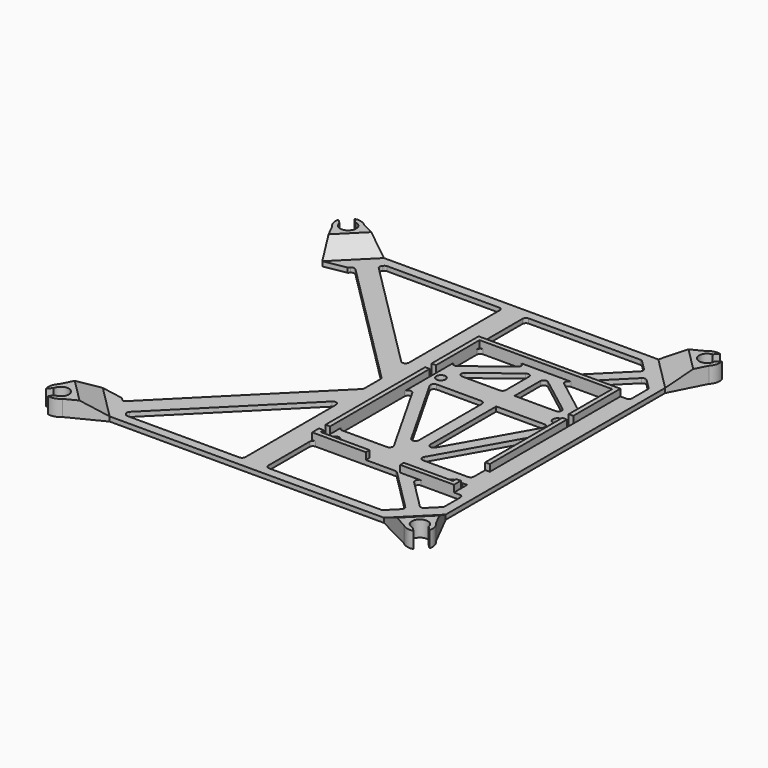
from build123d import *

# Parameters (mm, degrees)
F0_W          = 150
F0_H          = 150
F1_DEPTH      = 2
F2_W          = 62
F2_H          = 91
F2_W_2        = 58
F2_H_2        = 87
F3_DEPTH      = 3
F4_W          = 15
F4_H          = 2
F4_W_2        = 2
F4_H_2        = 14
F5_DEPTH      = 3
F6_R          = 2
F6_W          = 2
F6_H          = 3.5
F7_DEPTH      = 25
F9_DEPTH      = 5
F9_DEPTH_BACK = 2
F10_DEPTH     = 5
F11_DEPTH     = 5
F12_SIZE2     = 4.99999
F12_SIZE      = 9.99999
F12_2_SIZE2   = 4.99999
F12_2_SIZE    = 9.99999
F12_3_SIZE2   = 4.99999
F12_3_SIZE    = 9.99999
F12_4_SIZE2   = 4.99999
F12_4_SIZE    = 9.99999
F14_DEPTH     = 25
F16_DEPTH     = 25
F17_R         = 1.5
F18_R         = 1.5
F19_R         = 1.5
F21_R         = 1
F23_DEPTH     = 25
F25_DEPTH     = 25


# Not quite as in the source:
# - two fillets or chamfers of one size are made in one step
# - a fillet or chamfer is up to 0.001 mm smaller than in the source, because OpenCascade refuses the exact size


with BuildPart() as f1:
    # F0 (on Top) → F1 (new body)
    with BuildSketch(Plane.XY):
        Rectangle(F0_W, F0_H)
    extrude(amount=F1_DEPTH)

    # F2 (on face) → F3 (join)
    with BuildSketch(Plane.XY.offset(2)):
        with Locations((36, 0)):
            Rectangle(F2_W, F2_H)
        with Locations((36, 0)):
            Rectangle(F2_W_2, F2_H_2, mode=Mode.SUBTRACT)
    extrude(amount=F3_DEPTH)

    # F4 (on face) → F5 (cut)
    with BuildSketch(Plane.XY.offset(5)):
        with Locations((36, -44.5)):
            Rectangle(F4_W, F4_H)
        with Locations((66, -32.9)):
            Rectangle(F4_W_2, F4_H_2)
    extrude(amount=-F5_DEPTH, mode=Mode.SUBTRACT)

    # F6 (on face) → F7 (cut)
    with BuildSketch(Plane.XY.offset(5)):
        with Locations((61.5, -40)):
            Circle(F6_R)
        with Locations((61.5, 18)):
            Circle(F6_R)
        with Locations((66, -40)):
            Rectangle(F6_W, F6_H)
        with Locations((66, 18)):
            Rectangle(F6_W, F6_H)
        with Locations((6, -40)):
            Rectangle(F6_W, F6_H)
        with Locations((6, 18)):
            Rectangle(F6_W, F6_H)
        with Locations((10.5, 18)):
            Circle(F6_R)
        with Locations((10.5, -40)):
            Circle(F6_R)
    extrude(amount=-F7_DEPTH, mode=Mode.SUBTRACT)

    # F8 (on face) → F9 (join, two sides)
    with BuildSketch(Plane.XY.offset(2)) as f9_sk:
        with BuildLine():
            ThreePointArc((82.0110086434, 78.1219213469), (76.0606601718, 76.0606601718), (78.1219213469, 82.0110086434))
            Line((78.1219213469, 82.0110086434), (79.959038654, 83.8481259505))
            ThreePointArc((79.959038654, 83.8481259505), (77.1120291579, 83.8481259505), (74.6464466094, 82.4246212025))
            Line((74.6464466094, 82.4246212025), (60, 75))
            Line((60, 75), (75, 60))
            Line((75, 60), (82.4246212025, 74.6464466094))
            ThreePointArc((82.4246212025, 74.6464466094), (83.8481259505, 77.1120291579), (83.8481259505, 79.959038654))
            Line((83.8481259505, 79.959038654), (82.0110086434, 78.1219213469))
        make_face()
        with BuildLine():
            Line((-60, 75), (-74.6464466094, 82.4246212025))
            ThreePointArc((-74.6464466094, 82.4246212025), (-77.1120291579, 83.8481259505), (-79.959038654, 83.8481259505))
            Line((-79.959038654, 83.8481259505), (-78.1219213469, 82.0110086434))
            ThreePointArc((-78.1219213469, 82.0110086434), (-76.0606601718, 76.0606601718), (-82.0110086434, 78.1219213469))
            Line((-82.0110086434, 78.1219213469), (-83.8481259505, 79.959038654))
            ThreePointArc((-83.8481259505, 79.959038654), (-83.8481259505, 77.1120291579), (-82.4246212025, 74.6464466094))
            Line((-82.4246212025, 74.6464466094), (-75, 60))
            Line((-75, 60), (-60, 75))
        make_face()
        with BuildLine():
            Line((-75, -60), (-82.4246212025, -74.6464466094))
            ThreePointArc((-82.4246212025, -74.6464466094), (-83.8481259505, -77.1120291579), (-83.8481259505, -79.959038654))
            Line((-83.8481259505, -79.959038654), (-82.0110086434, -78.1219213469))
            ThreePointArc((-82.0110086434, -78.1219213469), (-76.0606601718, -76.0606601718), (-78.1219213469, -82.0110086434))
            Line((-78.1219213469, -82.0110086434), (-79.959038654, -83.8481259505))
            ThreePointArc((-79.959038654, -83.8481259505), (-77.1120291579, -83.8481259505), (-74.6464466094, -82.4246212025))
            Line((-74.6464466094, -82.4246212025), (-60, -75))
            Line((-60, -75), (-75, -60))
        make_face()
        with BuildLine():
            Line((60, -75), (74.6464466094, -82.4246212025))
            ThreePointArc((74.6464466094, -82.4246212025), (77.1120291579, -83.8481259505), (79.959038654, -83.8481259505))
            Line((79.959038654, -83.8481259505), (78.1219213469, -82.0110086434))
            ThreePointArc((78.1219213469, -82.0110086434), (76.0606601718, -76.0606601718), (82.0110086434, -78.1219213469))
            Line((82.0110086434, -78.1219213469), (83.8481259505, -79.959038654))
            ThreePointArc((83.8481259505, -79.959038654), (83.8481259505, -77.1120291579), (82.4246212025, -74.6464466094))
            Line((82.4246212025, -74.6464466094), (75, -60))
            Line((75, -60), (60, -75))
        make_face()
    extrude(amount=F9_DEPTH)
    extrude(f9_sk.sketch, amount=-F9_DEPTH_BACK)

    # F8 (on face) → F10 (join)
    with BuildSketch(Plane.XY.offset(2)):
        with BuildLine():
            ThreePointArc((82.0110086434, 78.1219213469), (76.0606601718, 76.0606601718), (78.1219213469, 82.0110086434))
            Line((78.1219213469, 82.0110086434), (79.959038654, 83.8481259505))
            ThreePointArc((79.959038654, 83.8481259505), (77.1120291579, 83.8481259505), (74.6464466094, 82.4246212025))
            Line((74.6464466094, 82.4246212025), (60, 75))
            Line((60, 75), (75, 60))
            Line((75, 60), (82.4246212025, 74.6464466094))
            ThreePointArc((82.4246212025, 74.6464466094), (83.8481259505, 77.1120291579), (83.8481259505, 79.959038654))
            Line((83.8481259505, 79.959038654), (82.0110086434, 78.1219213469))
        make_face()
        with BuildLine():
            Line((-60, 75), (-74.6464466094, 82.4246212025))
            ThreePointArc((-74.6464466094, 82.4246212025), (-77.1120291579, 83.8481259505), (-79.959038654, 83.8481259505))
            Line((-79.959038654, 83.8481259505), (-78.1219213469, 82.0110086434))
            ThreePointArc((-78.1219213469, 82.0110086434), (-76.0606601718, 76.0606601718), (-82.0110086434, 78.1219213469))
            Line((-82.0110086434, 78.1219213469), (-83.8481259505, 79.959038654))
            ThreePointArc((-83.8481259505, 79.959038654), (-83.8481259505, 77.1120291579), (-82.4246212025, 74.6464466094))
            Line((-82.4246212025, 74.6464466094), (-75, 60))
            Line((-75, 60), (-60, 75))
        make_face()
        with BuildLine():
            Line((-75, -60), (-82.4246212025, -74.6464466094))
            ThreePointArc((-82.4246212025, -74.6464466094), (-83.8481259505, -77.1120291579), (-83.8481259505, -79.959038654))
            Line((-83.8481259505, -79.959038654), (-82.0110086434, -78.1219213469))
            ThreePointArc((-82.0110086434, -78.1219213469), (-76.0606601718, -76.0606601718), (-78.1219213469, -82.0110086434))
            Line((-78.1219213469, -82.0110086434), (-79.959038654, -83.8481259505))
            ThreePointArc((-79.959038654, -83.8481259505), (-77.1120291579, -83.8481259505), (-74.6464466094, -82.4246212025))
            Line((-74.6464466094, -82.4246212025), (-60, -75))
            Line((-60, -75), (-75, -60))
        make_face()
        with BuildLine():
            Line((60, -75), (74.6464466094, -82.4246212025))
            ThreePointArc((74.6464466094, -82.4246212025), (77.1120291579, -83.8481259505), (79.959038654, -83.8481259505))
            Line((79.959038654, -83.8481259505), (78.1219213469, -82.0110086434))
            ThreePointArc((78.1219213469, -82.0110086434), (76.0606601718, -76.0606601718), (82.0110086434, -78.1219213469))
            Line((82.0110086434, -78.1219213469), (83.8481259505, -79.959038654))
            ThreePointArc((83.8481259505, -79.959038654), (83.8481259505, -77.1120291579), (82.4246212025, -74.6464466094))
            Line((82.4246212025, -74.6464466094), (75, -60))
            Line((75, -60), (60, -75))
        make_face()
    extrude(amount=F10_DEPTH)

    # F8 (on face) → F11 (join)
    with BuildSketch(Plane.XY.offset(2)):
        with BuildLine():
            ThreePointArc((82.0110086434, 78.1219213469), (76.0606601718, 76.0606601718), (78.1219213469, 82.0110086434))
            Line((78.1219213469, 82.0110086434), (79.959038654, 83.8481259505))
            ThreePointArc((79.959038654, 83.8481259505), (77.1120291579, 83.8481259505), (74.6464466094, 82.4246212025))
            Line((74.6464466094, 82.4246212025), (60, 75))
            Line((60, 75), (75, 60))
            Line((75, 60), (82.4246212025, 74.6464466094))
            ThreePointArc((82.4246212025, 74.6464466094), (83.8481259505, 77.1120291579), (83.8481259505, 79.959038654))
            Line((83.8481259505, 79.959038654), (82.0110086434, 78.1219213469))
        make_face()
        with BuildLine():
            Line((-60, 75), (-74.6464466094, 82.4246212025))
            ThreePointArc((-74.6464466094, 82.4246212025), (-77.1120291579, 83.8481259505), (-79.959038654, 83.8481259505))
            Line((-79.959038654, 83.8481259505), (-78.1219213469, 82.0110086434))
            ThreePointArc((-78.1219213469, 82.0110086434), (-76.0606601718, 76.0606601718), (-82.0110086434, 78.1219213469))
            Line((-82.0110086434, 78.1219213469), (-83.8481259505, 79.959038654))
            ThreePointArc((-83.8481259505, 79.959038654), (-83.8481259505, 77.1120291579), (-82.4246212025, 74.6464466094))
            Line((-82.4246212025, 74.6464466094), (-75, 60))
            Line((-75, 60), (-60, 75))
        make_face()
        with BuildLine():
            Line((-75, -60), (-82.4246212025, -74.6464466094))
            ThreePointArc((-82.4246212025, -74.6464466094), (-83.8481259505, -77.1120291579), (-83.8481259505, -79.959038654))
            Line((-83.8481259505, -79.959038654), (-82.0110086434, -78.1219213469))
            ThreePointArc((-82.0110086434, -78.1219213469), (-76.0606601718, -76.0606601718), (-78.1219213469, -82.0110086434))
            Line((-78.1219213469, -82.0110086434), (-79.959038654, -83.8481259505))
            ThreePointArc((-79.959038654, -83.8481259505), (-77.1120291579, -83.8481259505), (-74.6464466094, -82.4246212025))
            Line((-74.6464466094, -82.4246212025), (-60, -75))
            Line((-60, -75), (-75, -60))
        make_face()
        with BuildLine():
            Line((60, -75), (74.6464466094, -82.4246212025))
            ThreePointArc((74.6464466094, -82.4246212025), (77.1120291579, -83.8481259505), (79.959038654, -83.8481259505))
            Line((79.959038654, -83.8481259505), (78.1219213469, -82.0110086434))
            ThreePointArc((78.1219213469, -82.0110086434), (76.0606601718, -76.0606601718), (82.0110086434, -78.1219213469))
            Line((82.0110086434, -78.1219213469), (83.8481259505, -79.959038654))
            ThreePointArc((83.8481259505, -79.959038654), (83.8481259505, -77.1120291579), (82.4246212025, -74.6464466094))
            Line((82.4246212025, -74.6464466094), (75, -60))
            Line((75, -60), (60, -75))
        make_face()
    extrude(amount=F11_DEPTH)

    # F12 (size 10 and 5 in the source; OpenCascade refuses exactly that, so slightly less here)
    f12_edges = [f1.edges().sort_by_distance(p)[0] for p in [
        (-67.5, 67.5, 7),
    ]]
    f12_side = f1.faces().sort_by_distance((-72.538706, 72.538706, 7))[0]
    chamfer(f12_edges, length=F12_SIZE, length2=F12_SIZE2, reference=f12_side)

    # F12#2 (size 10 and 5 in the source; OpenCascade refuses exactly that, so slightly less here)
    f12_2_edges = [f1.edges().sort_by_distance(p)[0] for p in [
        (67.5, 67.5, 7),
    ]]
    f12_2_side = f1.faces().sort_by_distance((72.538706, 72.538706, 7))[0]
    chamfer(f12_2_edges, length=F12_2_SIZE, length2=F12_2_SIZE2, reference=f12_2_side)

    # F12#3 (size 10 and 5 in the source; OpenCascade refuses exactly that, so slightly less here)
    f12_3_edges = [f1.edges().sort_by_distance(p)[0] for p in [
        (67.5, -67.5, 7),
    ]]
    f12_3_side = f1.faces().sort_by_distance((72.538706, -72.538706, 7))[0]
    chamfer(f12_3_edges, length=F12_3_SIZE, length2=F12_3_SIZE2, reference=f12_3_side)

    # F12#4 (size 10 and 5 in the source; OpenCascade refuses exactly that, so slightly less here)
    f12_4_edges = [f1.edges().sort_by_distance(p)[0] for p in [
        (-67.5, -67.5, 7),
    ]]
    f12_4_side = f1.faces().sort_by_distance((-72.538706, -72.538706, 7))[0]
    chamfer(f12_4_edges, length=F12_4_SIZE, length2=F12_4_SIZE2, reference=f12_4_side)

    # F13 (on face) → F14 (cut)
    with BuildSketch(Plane.XY.offset(2)):
        with BuildLine():
            ThreePointArc((-7.5606601718, 18.8743686708), (-5.9259748515, 18.5492095438), (-5, 19.9350288425))
            Line((-5, 19.9350288425), (-5, 71))
            Line((-5, 71), (-56, 71))
            Line((-56, 71), (-56.7824855787, 70.2175144213))
            ThreePointArc((-56.7824855787, 70.2175144213), (-57.2218254069, 69.1568542495), (-56.7824855787, 68.0961940777))
            Line((-56.7824855787, 68.0961940777), (-7.5606601718, 18.8743686708))
        make_face()
        Polygon((56, 71), (5, 71), (5, 45.5), (41.9644660941, 45.5), (61.732233047, 65.267766953), align=None)
        Polygon((67, -45.5), (49.0355339059, -45.5), (65.267766953, -61.732233047), (71, -56), (71, -45.5), align=None)
        Polygon((-5, -71), (-5, -16.313708499), (-57.8431457505, -69.1568542495), (-56, -71), align=None)
        Polygon((41.9644660941, -45.5), (5, -45.5), (5, -71), (56, -71), (61.732233047, -65.267766953), align=None)
        Polygon((-65.267766953, 61.732233047), (-71, 56), (-71, 5), (-71, -5), (-5, -5), (-5, 5), (-63.5, 63.5), align=None)
        Polygon((-5, -5), (-71, -5), (-71, -56), (-65.267766953, -61.732233047), (-63.5, -63.5), align=None)
        Polygon((65.267766953, 61.732233047), (49.0355339059, 45.5), (67, 45.5), (71, 45.5), (71, 56), align=None)
    extrude(amount=-F14_DEPTH, mode=Mode.SUBTRACT)

    # F15 (on face) → F16 (cut)
    with BuildSketch(Plane.XY.offset(5)):
        with BuildLine():
            Line((33.5, -22.7423213834), (33.5, 11.75))
            ThreePointArc((33.5, 11.75), (33.0606601718, 12.8106601718), (32, 13.25))
            Line((32, 13.25), (12.4482028522, 13.25))
            ThreePointArc((12.4482028522, 13.25), (11.1521429804, 12.5051349607), (11.1432693585, 11.0103050784))
            Line((11.1432693585, 11.0103050784), (30.6950665063, -23.482016305))
            ThreePointArc((30.6950665063, -23.482016305), (32.3824916727, -24.1927351589), (33.5, -22.7423213834))
        make_face()
        with BuildLine():
            ThreePointArc((25.8598739427, 40.808144173), (26.3699933362, 42.4807370692), (24.949116188, 43.5))
            Line((24.949116188, 43.5), (8.5, 43.5))
            ThreePointArc((8.5, 43.5), (7.4393398282, 43.0606601718), (7, 42))
            Line((7, 42), (7, 29.4303923469))
            ThreePointArc((7, 29.4303923469), (7.8352205749, 28.0857480385), (9.4107577546, 28.2385365198))
            Line((9.4107577546, 28.2385365198), (25.8598739427, 40.808144173))
        make_face()
        with BuildLine():
            ThreePointArc((60.8567306415, 11.0103050784), (60.8478570196, 12.5051349607), (59.5517971478, 13.25))
            Line((59.5517971478, 13.25), (40, 13.25))
            ThreePointArc((40, 13.25), (38.9393398282, 12.8106601718), (38.5, 11.75))
            Line((38.5, 11.75), (38.5, -22.7423213834))
            ThreePointArc((38.5, -22.7423213834), (39.6175083273, -24.1927351589), (41.3049334937, -23.482016305))
            Line((41.3049334937, -23.482016305), (60.8567306415, 11.0103050784))
        make_face()
        with BuildLine():
            ThreePointArc((33.5, 37.3196076531), (32.6647794251, 38.6642519615), (31.0892422454, 38.5114634802))
            Line((31.0892422454, 38.5114634802), (14.6401260573, 25.941855827))
            ThreePointArc((14.6401260573, 25.941855827), (14.1300066638, 24.2692629308), (15.550883812, 23.25))
            Line((15.550883812, 23.25), (32, 23.25))
            ThreePointArc((32, 23.25), (33.0606601718, 23.6893398282), (33.5, 24.75))
            Line((33.5, 24.75), (33.5, 37.3196076531))
        make_face()
        with BuildLine():
            Line((65, -25.9), (65, 2.4923213834))
            ThreePointArc((65, 2.4923213834), (63.8824916727, 3.9427351589), (62.1950665063, 3.232016305))
            Line((62.1950665063, 3.232016305), (42.6432693585, -31.2603050784))
            ThreePointArc((42.6432693585, -31.2603050784), (42.6521429804, -32.7551349607), (43.9482028522, -33.5))
            Line((43.9482028522, -33.5), (63.5, -33.5))
            ThreePointArc((63.5, -33.5), (64.5606601718, -33.0606601718), (65, -32))
            Line((65, -32), (65, -25.9))
        make_face()
        with BuildLine():
            ThreePointArc((40, 23.25), (38.9393398282, 23.6893398282), (38.5, 24.75))
            Line((38.5, 24.75), (38.5, 23.25))
            Line((38.5, 23.25), (40, 23.25))
        make_face()
        with BuildLine():
            Line((63.5, 43.5), (47.050883812, 43.5))
            ThreePointArc((47.050883812, 43.5), (45.6300066638, 42.4807370692), (46.1401260573, 40.808144173))
            Line((46.1401260573, 40.808144173), (62.5892422454, 28.2385365198))
            ThreePointArc((62.5892422454, 28.2385365198), (64.1647794251, 28.0857480385), (65, 29.4303923469))
            Line((65, 29.4303923469), (65, 42))
            ThreePointArc((65, 42), (64.5606601718, 43.0606601718), (63.5, 43.5))
        make_face()
        with BuildLine():
            ThreePointArc((9.8049334937, 3.232016305), (8.1175083273, 3.9427351589), (7, 2.4923213834))
            Line((7, 2.4923213834), (7, -32))
            ThreePointArc((7, -32), (7.4393398282, -33.0606601718), (8.5, -33.5))
            Line((8.5, -33.5), (28.0517971478, -33.5))
            ThreePointArc((28.0517971478, -33.5), (29.3478570196, -32.7551349607), (29.3567306415, -31.2603050784))
            Line((29.3567306415, -31.2603050784), (9.8049334937, 3.232016305))
        make_face()
        with BuildLine():
            ThreePointArc((38.5, 11.75), (38.9393398282, 12.8106601718), (40, 13.25))
            Line((40, 13.25), (38.5, 13.25))
            Line((38.5, 13.25), (38.5, 11.75))
        make_face()
        with BuildLine():
            ThreePointArc((40.9107577546, 38.5114634802), (39.3352205749, 38.6642519615), (38.5, 37.3196076531))
            Line((38.5, 37.3196076531), (38.5, 24.75))
            ThreePointArc((38.5, 24.75), (38.9393398282, 23.6893398282), (40, 23.25))
            Line((40, 23.25), (56.449116188, 23.25))
            ThreePointArc((56.449116188, 23.25), (57.8699933362, 24.2692629308), (57.3598739427, 25.941855827))
            Line((57.3598739427, 25.941855827), (40.9107577546, 38.5114634802))
        make_face()
    extrude(amount=-F16_DEPTH, mode=Mode.SUBTRACT)

    # F17
    f17_edges = [f1.edges().sort_by_distance(p)[0] for p in [
        (-56, 71, 1),
    ]]
    fillet(f17_edges, radius=F17_R)

    # F18
    f18_edges = [f1.edges().sort_by_distance(p)[0] for p in [
        (-5, 71, 1),
        (-63.5, 63.5, 1),
        (-56, -71, 1),
        (-57.843146, -69.156854, 1),
        (-5, -16.313708, 1),
        (-5, -71, 1),
        (41.964466, -45.5, 1),
        (61.732233, -65.267767, 1),
        (56, -71, 1),
        (5, -45.5, 1),
        (5, -71, 1),
        (71, -56, 1),
        (65.267767, -61.732233, 1),
        (49.035534, -45.5, 1),
        (71, -45.5, 1),
        (-5, -5, 1),
        (56, 71, 1),
        (61.732233, 65.267767, 1),
        (41.964466, 45.5, 1),
        (5, 71, 1),
        (5, 45.5, 1),
        (49.035534, 45.5, 1),
        (71, 45.5, 1),
        (65.267767, 61.732233, 1),
        (71, 56, 1),
    ]]
    fillet(f18_edges, radius=F18_R)

    # F19
    f19_edges = [f1.edges().sort_by_distance(p)[0] for p in [
        (-71, 56, 1),
        (-71, -56, 1),
    ]]
    fillet(f19_edges, radius=F19_R)

    # F21
    f21_edges = [f1.edges().sort_by_distance(p)[0] for p in [
        (-5, 5, 1),
        (-63.5, -63.5, 1),
    ]]
    fillet(f21_edges, radius=F21_R)

    # F22 (on face) → F23 (cut)
    with BuildSketch(Plane.XY.offset(2)):
        Polygon((-71, 56), (-75, 60), (-75, -60), (-71, -56), align=None)
    extrude(amount=-F23_DEPTH, mode=Mode.SUBTRACT)

    # F24 (on face) → F25 (cut)
    with BuildSketch(Plane.XY.offset(2)):
        Polygon((-75, -60), (-65.267766953, -61.732233047), (-72.2899705172, -52.5203099847), align=None)
        Polygon((-75, 60), (-72.2899705172, 52.5203099847), (-65.267766953, 61.732233047), align=None)
    extrude(amount=-F25_DEPTH, mode=Mode.SUBTRACT)


solid = f1.part
